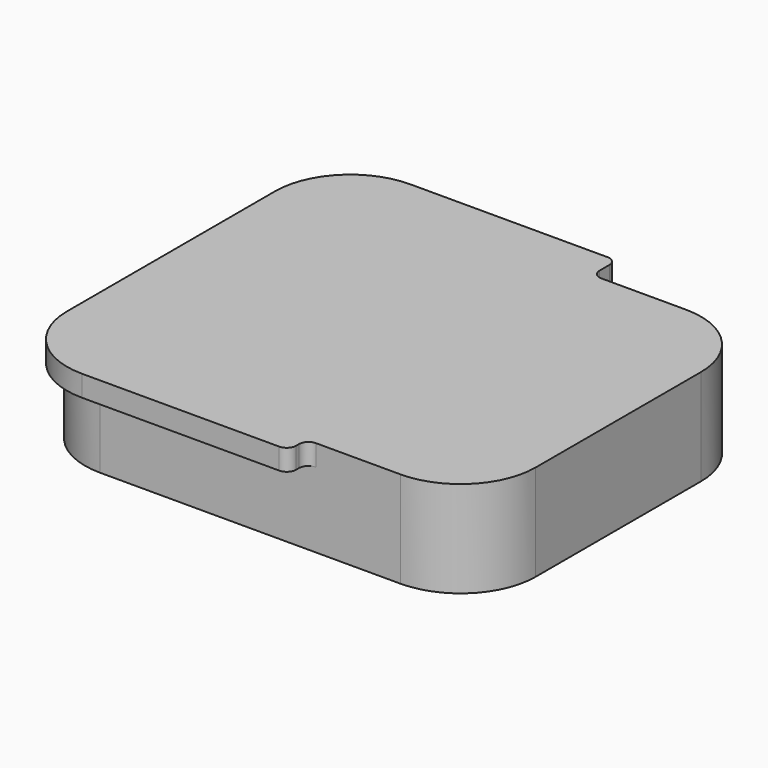
from build123d import *

# Parameters (mm, degrees)
F1_DEPTH     = 10.25
F3_DEPTH     = 2.25
F4_R         = 1
F5_T         = 1.9
F5_T3_DEPTH  = 4.8
F5_T5_DEPTH  = 25.8
F5_T8_ANGLE  = 90.000000001
F5_T10_ANGLE = 90.000000001
F7_DEPTH     = 2.25
F9_DEPTH     = 6.4


# Not quite as in the source:
# - a shell that OpenCascade refuses in one call is made with other operations: the cavity is built on its own and cut out


with BuildPart() as f1:
    # F0 (on Top) → F1 (new body)
    with BuildSketch(Plane.XY):
        with BuildLine():
            Line((16, 19), (-16, 19))
            ThreePointArc((-16, 19), (-21.6568542495, 16.6568542495), (-24, 11))
            Line((-24, 11), (-24, -11))
            ThreePointArc((-24, -11), (-21.6568542495, -16.6568542495), (-16, -19))
            Line((-16, -19), (16, -19))
            ThreePointArc((16, -19), (21.6568542495, -16.6568542495), (24, -11))
            Line((24, -11), (24, 11))
            ThreePointArc((24, 11), (21.6568542495, 16.6568542495), (16, 19))
        make_face()
    extrude(amount=F1_DEPTH)

    # F2 (on face) → F3 (join)
    with BuildSketch(Plane.XY.offset(10.25)):
        with BuildLine():
            Line((6, 22.309198174), (-16, 22.309198174))
            ThreePointArc((-16, 22.309198174), (-21.6568542495, 19.9660524235), (-24, 14.309198174))
            Line((-24, 14.309198174), (-24, 11))
            ThreePointArc((-24, 11), (-21.6568542495, 16.6568542495), (-16, 19))
            Line((-16, 19), (6, 19))
            Line((6, 19), (6, 22.309198174))
        make_face()
        with BuildLine():
            Line((6, -21.390801826), (6, -19))
            Line((6, -19), (-16, -19))
            ThreePointArc((-16, -19), (-21.6568542495, -16.6568542495), (-24, -11))
            Line((-24, -11), (-24, -13.390801826))
            ThreePointArc((-24, -13.390801826), (-21.6568542495, -19.0476560755), (-16, -21.390801826))
            Line((-16, -21.390801826), (6, -21.390801826))
        make_face()
    extrude(amount=-F3_DEPTH)

    # F4
    f4_edges = [f1.edges().sort_by_distance(p)[0] for p in [
        (6, -21.390802, 9.125),
        (6, -19, 9.125),
        (6, 19, 9.125),
        (6, 22.309198, 9.125),
    ]]
    fillet(f4_edges, radius=F4_R)

    # F5: shell of thickness 1.9, made by hand


with BuildPart() as f5_core1:
    # F5_t2: copy of F1
    add(f1.part)

    # the walls: a layer under each face that stays
    f5_faces = [f5_core1.faces().sort_by_distance(p)[0] for p in [
        (0, 19, 5.125),
        (0, 0.459198174, 10.25),
        (6.2928932188, 19.2928932188, 9.125),
        (21.6568542495, 16.6568542495, 5.125),
        (-18.8333333333, 20.4243318117, 8),
        (-21.6568542495, 16.6568542495, 4),
        (6, 20.654599087, 9.125),
        (24, 0, 5.125),
        (21.6568542495, -16.6568542495, 5.125),
        (-5.5, 22.309198174, 9.125),
        (0, -19, 5.125),
        (-21.6568542495, 19.9660524235, 9.125),
        (6.2928932188, -19.2928932188, 9.125),
        (-24, 0.459198174, 5.125),
        (6, -20.195400913, 9.125),
        (-21.6568542495, -19.0476560755, 9.125),
        (-5.5, -21.390801826, 9.125),
        (-21.6568542495, -16.6568542495, 4),
        (-18.8333333333, -19.6590015216, 8),
    ]]
    thicken(f5_faces, amount=-F5_T, mode=Mode.SUBTRACT)

    # F5_s4 → F5_t3 (cut)
    with BuildSketch(Plane.YZ.offset(4.1)):
        Polygon((19.019, 7.981), (17.1, 8), (17.1, 9.9), (19, 9.9), align=None)
        Polygon((-19.019, 7.981), (-17.1, 8), (-17.1, 9.9), (-19, 9.9), align=None)
    extrude(amount=F5_T3_DEPTH, mode=Mode.SUBTRACT)

    # F5_s6 → F5_t5 (cut)
    with BuildSketch(Plane.YZ.offset(-17.9)):
        Polygon((19.019, 7.981), (17.1, 8), (17.1, 9.9), (19, 9.9), align=None)
        Polygon((-19.019, 7.981), (-17.1, 8), (-17.1, 9.9), (-19, 9.9), align=None)
    extrude(amount=F5_T5_DEPTH, mode=Mode.SUBTRACT)

    # F5_s7 → F5_t8 (revolve, cut)
    with BuildSketch(Plane.XZ.offset(-11)):
        Polygon((-24.019, 7.981), (-24, 9.9), (-22.1, 9.9), (-22.1, 8), align=None)
    revolve(axis=Axis((-16, 11, 8), (0, 0, -1)), revolution_arc=F5_T8_ANGLE, mode=Mode.SUBTRACT)

    # F5_s9 → F5_t10 (revolve, cut)
    with BuildSketch(Plane.YZ.offset(-16)):
        Polygon((-19.019, 7.981), (-17.1, 8), (-17.1, 9.9), (-19, 9.9), align=None)
    revolve(axis=Axis((-16, -11, 8), (0, 0, -1)), revolution_arc=F5_T10_ANGLE, mode=Mode.SUBTRACT)


with BuildPart() as f1_1:
    add(f1.part)

    # what is left inside the walls is the cavity
    f5_cavity = [f5_core1.part.solids().sort_by_distance(p)[0] for p in [
        (0, -5.7, 0.019),
    ]]
    add(f5_cavity, mode=Mode.SUBTRACT)

    # F6 (on face) → F7 (cut)
    with BuildSketch(Plane(origin=(0, 0, 0), x_dir=(1, 0, 0), z_dir=(0, 0, -1))):
        with BuildLine():
            ThreePointArc((-16, 18.1000009179), (-21.0204587955, 16.0204587955), (-23.1000009179, 11))
            Line((-23.1000009179, 11), (-23.1000009179, -11))
            ThreePointArc((-23.1000009179, -11), (-21.0204587955, -16.0204587955), (-16, -18.1000009179))
            Line((-16, -18.1000009179), (16, -18.1000009179))
            ThreePointArc((16, -18.1000009179), (21.0204587955, -16.0204587955), (23.1000009179, -11))
            Line((23.1000009179, -11), (23.1000009179, 11))
            ThreePointArc((23.1000009179, 11), (21.0204587955, 16.0204587955), (16, 18.1000009179))
            Line((16, 18.1000009179), (-16, 18.1000009179))
        make_face()
        with BuildLine():
            Line((16, -17.1), (-16, -17.1))
            ThreePointArc((-16, -17.1), (-20.3133513652, -15.3133513652), (-22.1, -11))
            Line((-22.1, -11), (-22.1, 11))
            ThreePointArc((-22.1, 11), (-20.3133513652, 15.3133513652), (-16, 17.1))
            Line((-16, 17.1), (16, 17.1))
            ThreePointArc((16, 17.1), (20.3133513652, 15.3133513652), (22.1, 11))
            Line((22.1, 11), (22.1, -11))
            ThreePointArc((22.1, -11), (20.3133513652, -15.3133513652), (16, -17.1))
        make_face(mode=Mode.SUBTRACT)
    extrude(amount=-F7_DEPTH, mode=Mode.SUBTRACT)

    # F8 (on face) → F9 (cut)
    with BuildSketch(Plane(origin=(-24, 0, 0), x_dir=(0, -1, 0), z_dir=(-1, 0, 0))):
        with BuildLine():
            Line((-5.5, 0), (5.5, 0))
            ThreePointArc((5.5, 0), (0, 5.5), (-5.5, 0))
        make_face()
    extrude(amount=-F9_DEPTH, mode=Mode.SUBTRACT)


solid = f1_1.part
